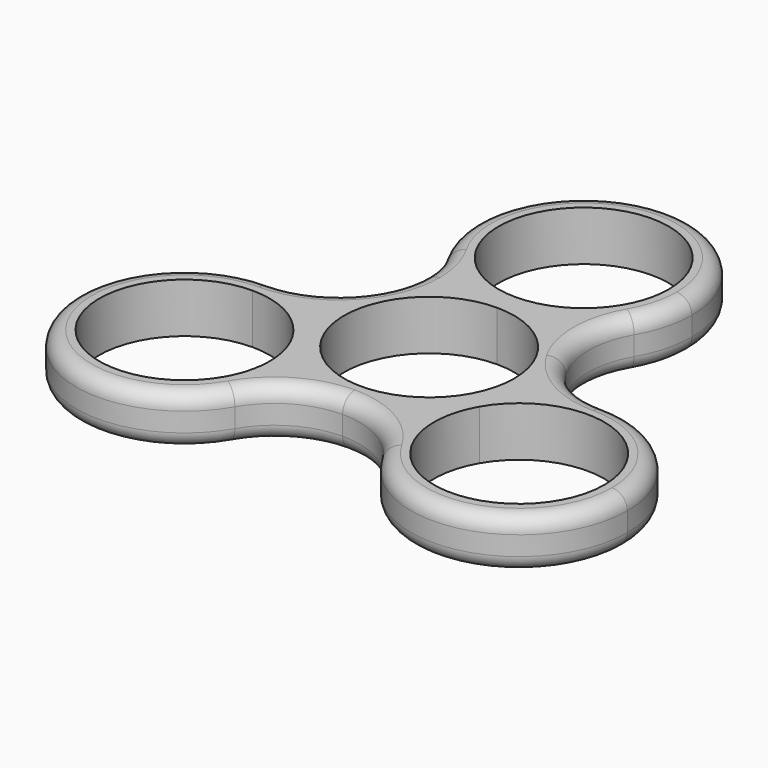
from build123d import *

# Parameters (mm, degrees)
F1_DEPTH = 6.5
F2_R     = 2


# Not quite as in the source:
# - ends of sketch curves that miss each other by under 0.0002 mm in the source are joined


with BuildPart() as f1:
    # F0 (on Top) → F1 (new body)
    with BuildSketch(Plane.XY):
        with BuildLine():
            Line((-12.2109581934, 18.15), (-9.612881982, 19.65))
            ThreePointArc((-9.612881982, 19.65), (-2.8728914006, 35.9217766718), (11.1, 25.2))
            ThreePointArc((11.1, 25.2), (10.7217766718, 22.3271085994), (9.612881982, 19.65))
            Line((9.612881982, 19.65), (12.2109581934, 18.15))
            ThreePointArc((12.2109581619, 18.1499999455), (13.6195541425, 21.5506514337), (14.1, 25.2))
            ThreePointArc((14.1, 25.2), (-3.649348519, 38.8195541552), (-12.2109582109, 18.1500000304))
        make_face()
        with BuildLine():
            ThreePointArc((-6.3285069329, 12.6), (-3.2519225117, 13.7198760919), (-7e-09, 14.1))
            ThreePointArc((-7e-09, 14.1), (-5.550000003, 15.5871180197), (-9.612881982, 19.65))
            Line((-9.612881982, 19.65), (-12.2109581934, 18.15))
            ThreePointArc((-12.2109582109, 18.1500000304), (-9.6761855625, 14.9442000331), (-6.3285069329, 12.6))
        make_face()
        with BuildLine():
            ThreePointArc((-12.2109580547, 7.0500002402), (-9.6761854488, 10.2558000741), (-6.3285069329, 12.6))
            ThreePointArc((-6.3285069329, 12.6), (-9.6761855625, 14.9442000331), (-12.2109582109, 18.1500000304))
            ThreePointArc((-12.2109582109, 18.1500000304), (-11.1020635081, 15.4728914176), (-10.7238401754, 12.6))
            ThreePointArc((-10.7238401754, 12.6), (-11.1020634677, 9.7271087333), (-12.2109580547, 7.0500002402))
        make_face()
        with BuildLine():
            ThreePointArc((-9.6128816287, -5.5500006119), (-9.6128821611, 5.5499996898), (-9.7e-09, 11.1))
            ThreePointArc((-9.7e-09, 11.1), (-3.251922513, 11.4801239084), (-6.3285069329, 12.6))
            ThreePointArc((-6.3285069329, 12.6), (-9.6761854488, 10.2558000741), (-12.2109580547, 7.0500002402))
            ThreePointArc((-12.2109580547, 7.0500002402), (-13.7198760608, 3.2519226432), (-14.0761735541, -0.8193522281))
            ThreePointArc((-14.0761735541, -0.8193522281), (-11.568039954, -2.9238147073), (-9.6128816287, -5.5500006119))
        make_face()
        with BuildLine():
            ThreePointArc((-21.8238401754, 1.5), (-17.7801496323, 0.9077224872), (-14.0761735541, -0.8193522281))
            ThreePointArc((-14.0761735541, -0.8193522281), (-13.7198760608, 3.2519226432), (-12.2109580547, 7.0500002402))
            ThreePointArc((-12.2109580547, 7.0500002402), (-16.2738400553, 2.9871180873), (-21.8238401754, 1.5))
        make_face()
        with BuildLine():
            ThreePointArc((-12.2109580547, -7.0500002402), (-13.5077224475, -4.0436906759), (-14.0761735541, -0.8193522281))
            ThreePointArc((-14.0761735541, -0.8193522281), (-17.7801496323, 0.9077224872), (-21.8238401754, 1.5))
            Line((-21.8238401754, 1.5), (-21.8238401754, -1.5))
            ThreePointArc((-21.8238401754, -1.5), (-16.2738400553, -2.9871180873), (-12.2109580547, -7.0500002402))
        make_face()
        with BuildLine():
            Line((-21.8238401754, -1.5), (-21.8238401754, 1.5))
            ThreePointArc((-21.8238401754, 1.5), (-34.0347983948, -19.6499999548), (-9.6128820342, -19.6500000904))
            Line((-9.6128820342, -19.6500000904), (-12.2109581934, -18.15))
            ThreePointArc((-12.2109581934, -18.15), (-31.4367221574, -18.15), (-21.8238401754, -1.5))
        make_face()
        with BuildLine():
            ThreePointArc((-7.7238401754, -12.6), (-7.7297980456, -12.1901507066), (-7.7476666212, -11.7806477719))
            ThreePointArc((-7.7476666212, -11.7806477719), (-10.2557998838, -9.6761856506), (-12.2109580547, -7.0500002402))
            ThreePointArc((-12.2109580547, -7.0500002402), (-11.1020634677, -9.7271087333), (-10.7238401754, -12.6))
            ThreePointArc((-10.7238401754, -12.6), (-11.1020635036, -15.4728914006), (-12.2109581934, -18.15))
            Line((-12.2109581934, -18.15), (-9.612881982, -19.65))
            ThreePointArc((-9.612881982, -19.65), (-8.2042860382, -16.2493485864), (-7.7238401754, -12.6))
        make_face()
        with BuildLine():
            ThreePointArc((-7.7476666212, -11.7806477719), (-8.3161175868, -8.5563097954), (-9.6128816287, -5.5500006119))
            ThreePointArc((-9.6128816287, -5.5500006119), (-11.568039954, -2.9238147073), (-14.0761735541, -0.8193522281))
            ThreePointArc((-14.0761735541, -0.8193522281), (-13.5077224475, -4.0436906759), (-12.2109580547, -7.0500002402))
            ThreePointArc((-12.2109580547, -7.0500002402), (-10.2557998838, -9.6761856506), (-7.7476666212, -11.7806477719))
        make_face()
        with BuildLine():
            ThreePointArc((0, -14.1), (-4.043690543, -13.5077224872), (-7.7476666212, -11.7806477719))
            ThreePointArc((-7.7476666212, -11.7806477719), (-7.7297980456, -12.1901507066), (-7.7238401754, -12.6))
            ThreePointArc((-7.7238401754, -12.6), (-8.2042860382, -16.2493485864), (-9.6128820342, -19.6500000904))
            ThreePointArc((-9.6128820342, -19.6500000904), (-5.5500000452, -15.5871180441), (0, -14.1))
        make_face()
        with BuildLine():
            ThreePointArc((7.7476666212, -11.7806477719), (8.3161176063, -8.5563097302), (9.6128816968, -5.550000494))
            ThreePointArc((9.6128816968, -5.550000494), (6.81e-08, -11.1), (-9.6128816287, -5.5500006119))
            ThreePointArc((-9.6128816287, -5.5500006119), (-8.3161175868, -8.5563097954), (-7.7476666212, -11.7806477719))
            ThreePointArc((-7.7476666212, -11.7806477719), (-4.043690543, -13.5077224872), (0, -14.1))
            ThreePointArc((0, -14.1), (4.043690543, -13.5077224872), (7.7476666212, -11.7806477719))
        make_face()
        with BuildLine():
            ThreePointArc((9.6128819758, -19.6499999892), (8.1039640812, -15.8519225022), (7.7476666212, -11.7806477719))
            ThreePointArc((7.7476666212, -11.7806477719), (4.043690543, -13.5077224872), (0, -14.1))
            ThreePointArc((0, -14.1), (5.5499999946, -15.5871180149), (9.6128819758, -19.6499999892))
        make_face()
        with BuildLine():
            ThreePointArc((12.2109582009, -7.0499999869), (10.2557999841, -9.6761855442), (7.7476666212, -11.7806477719))
            ThreePointArc((7.7476666212, -11.7806477719), (8.1039640812, -15.8519225022), (9.6128819758, -19.6499999892))
            Line((9.612881982, -19.65), (12.2109581934, -18.15))
            ThreePointArc((12.2109581934, -18.15), (10.7238401754, -12.5999999925), (12.2109582009, -7.0499999869))
        make_face()
        with BuildLine():
            ThreePointArc((14.0761735541, -0.8193522281), (11.5680400007, -2.9238146578), (9.6128816968, -5.550000494))
            ThreePointArc((9.6128816968, -5.550000494), (8.3161176063, -8.5563097302), (7.7476666212, -11.7806477719))
            ThreePointArc((7.7476666212, -11.7806477719), (10.2557999841, -9.6761855442), (12.2109582009, -7.0499999869))
            ThreePointArc((12.2109582009, -7.0499999869), (13.5077224894, -4.0436905358), (14.0761735541, -0.8193522281))
        make_face()
        with BuildLine():
            ThreePointArc((21.8238401754, 1.5), (17.7801496323, 0.9077224872), (14.0761735541, -0.8193522281))
            ThreePointArc((14.0761735541, -0.8193522281), (13.5077224894, -4.0436905358), (12.2109582009, -7.0499999869))
            ThreePointArc((12.2109582009, -7.0499999869), (16.2738401819, -2.9871180142), (21.8238401754, -1.5))
            Line((21.8238401754, -1.5), (21.8238401754, 1.5))
        make_face()
        with BuildLine():
            ThreePointArc((35.9238401754, -12.6), (31.7940457901, -2.6297943853), (21.8238401754, 1.5))
            Line((21.8238401754, 1.5), (21.8238401754, -1.5))
            ThreePointArc((21.8238401754, -1.5), (29.6727254465, -4.7511147288), (32.9238401754, -12.6))
            ThreePointArc((32.9238401754, -12.6), (24.696731576, -23.3217766718), (12.2109581934, -18.15))
            Line((12.2109581934, -18.15), (9.612881982, -19.65))
            ThreePointArc((9.6128819758, -19.6499999892), (25.4731887053, -26.2195541523), (35.9238401754, -12.6))
        make_face()
        with BuildLine():
            ThreePointArc((14.1, 0), (14.0940421298, -0.4098492934), (14.0761735541, -0.8193522281))
            ThreePointArc((14.0761735541, -0.8193522281), (17.7801496323, 0.9077224872), (21.8238401754, 1.5))
            ThreePointArc((21.8238401754, 1.5), (16.2738401733, 2.9871180192), (12.210958191, 7.0500000041))
            ThreePointArc((12.210958191, 7.0500000041), (13.6195541501, 3.6493485383), (14.1, 0))
        make_face()
        with BuildLine():
            ThreePointArc((-9.7e-09, 11.1), (7.8488852677, 7.8488852746), (11.1, 0))
            ThreePointArc((11.1, 0), (10.721776598, -2.8728916761), (9.6128816968, -5.550000494))
            ThreePointArc((9.6128816968, -5.550000494), (11.5680400007, -2.9238146578), (14.0761735541, -0.8193522281))
            ThreePointArc((14.0761735541, -0.8193522281), (14.0940421298, -0.4098492934), (14.1, 0))
            ThreePointArc((14.1, 0), (13.6195541501, 3.6493485383), (12.210958191, 7.0500000041))
            ThreePointArc((12.210958191, 7.0500000041), (9.676185548, 10.2557999806), (6.3285069329, 12.6))
            ThreePointArc((6.3285069329, 12.6), (3.2519225036, 11.4801239061), (-9.7e-09, 11.1))
        make_face()
        with BuildLine():
            ThreePointArc((12.2109581619, 18.1499999455), (9.6761855268, 14.9441999995), (6.3285069329, 12.6))
            ThreePointArc((6.3285069329, 12.6), (9.676185548, 10.2557999806), (12.210958191, 7.0500000041))
            ThreePointArc((12.210958191, 7.0500000041), (10.7238401754, 12.5999999709), (12.2109581619, 18.1499999455))
        make_face()
        with BuildLine():
            ThreePointArc((9.612881982, 19.65), (5.549999997, 15.5871180162), (-7e-09, 14.1))
            ThreePointArc((-7e-09, 14.1), (3.2519225049, 13.7198760935), (6.3285069329, 12.6))
            ThreePointArc((6.3285069329, 12.6), (9.6761855268, 14.9441999995), (12.2109581619, 18.1499999455))
            Line((12.2109581934, 18.15), (9.612881982, 19.65))
        make_face()
        with BuildLine():
            Line((0, 14.1), (0, 11.1))
            ThreePointArc((-9.7e-09, 11.1), (3.2519225036, 11.4801239061), (6.3285069329, 12.6))
            ThreePointArc((6.3285069329, 12.6), (3.2519225049, 13.7198760935), (-7e-09, 14.1))
        make_face()
        with BuildLine():
            ThreePointArc((-6.3285069329, 12.6), (-3.251922513, 11.4801239084), (-9.7e-09, 11.1))
            Line((0, 11.1), (0, 14.1))
            ThreePointArc((-7e-09, 14.1), (-3.2519225117, 13.7198760919), (-6.3285069329, 12.6))
        make_face()
    extrude(amount=F1_DEPTH)

    # F2
    f2_edges = [f1.edges().sort_by_distance(p)[0] for p in [
        (0, -14.1, 6.5),
        (0, -14.1, 0),
        (12.210958, 7.05, 0),
        (12.210958, 7.05, 6.5),
        (0, 39.3, 0),
        (0, 39.3, 6.5),
        (-12.210958, 7.05, 0),
        (-12.210958, 7.05, 6.5),
        (-34.034798, -19.65, 0),
        (-34.034798, -19.65, 6.5),
        (34.034798, -19.65, 0),
        (34.034798, -19.65, 6.5),
    ]]
    fillet(f2_edges, radius=F2_R)


solid = f1.part
